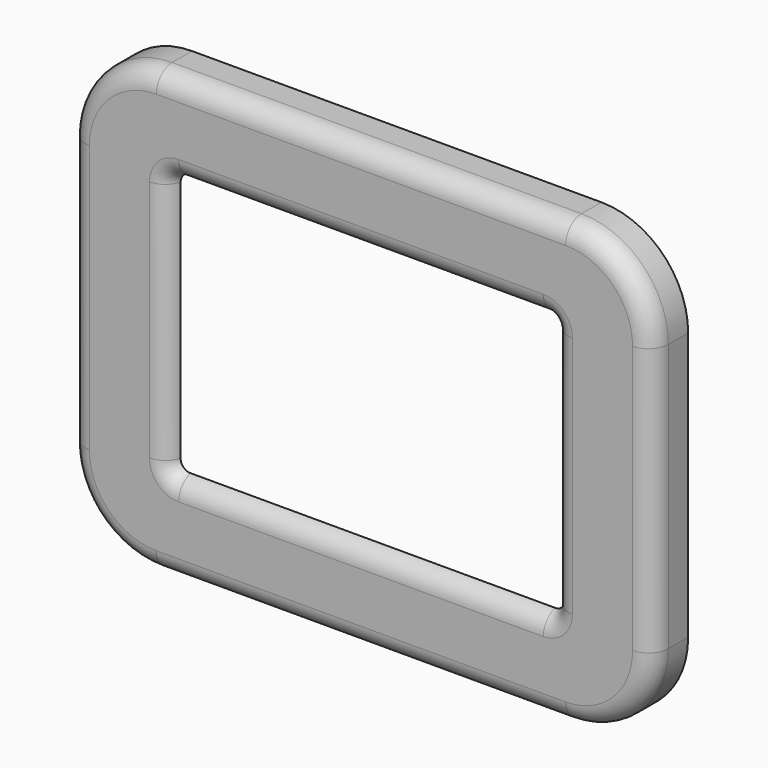
from build123d import *

# Parameters (mm, degrees)
F0_W         = 235
F0_H         = 178
F0_W_2       = 207
F0_H_2       = 156
F0_W_3       = 155
F0_H_3       = 106
F1_DEPTH     = 18
F2_DEPTH     = 12
F3_R         = 35
F4_R         = 4
F5_T1_DEPTH  = 98
F5_T3_DEPTH  = 147
F5_T5_DEPTH  = 165
F5_T7_DEPTH  = 108
F5_T10_ANGLE = 90
F5_T12_ANGLE = 90
F5_T14_ANGLE = 90
F5_T16_ANGLE = 90
F5_T18_ANGLE = 90
F5_T20_ANGLE = 90
F5_T22_ANGLE = 90
F5_T24_ANGLE = 90
F6_SIZE      = 3
F7_R         = 1.5
F8_DEPTH     = 16


# Not quite as in the source:
# - a fillet or chamfer that OpenCascade refuses, or shapes differently, is made with other operations: its cross-section is extruded or revolved along the edge and cut away or added


with BuildPart() as f1:
    # F0 (on Front) → F1 (new body)
    with BuildSketch(Plane.XZ):
        Rectangle(F0_W, F0_H)
        Rectangle(F0_W_2, F0_H_2, mode=Mode.SUBTRACT)
        Rectangle(F0_W_2, F0_H_2)
        Rectangle(F0_W_3, F0_H_3, mode=Mode.SUBTRACT)
    extrude(amount=F1_DEPTH)

    # F0 (on Front) → F2 (cut)
    with BuildSketch(Plane.XZ):
        Rectangle(F0_W_2, F0_H_2)
        Rectangle(F0_W_3, F0_H_3, mode=Mode.SUBTRACT)
    extrude(amount=F2_DEPTH, mode=Mode.SUBTRACT)

    # F3
    f3_edges = [f1.edges().sort_by_distance(p)[0] for p in [
        (117.5, -9, 89),
        (-117.5, -9, 89),
        (117.5, -9, -89),
        (-117.5, -9, -89),
    ]]
    fillet(f3_edges, radius=F3_R)

    # F4
    f4_edges = [f1.edges().sort_by_distance(p)[0] for p in [
        (-77.5, -15, 53),
        (77.5, -15, 53),
        (77.5, -15, -53),
        (-77.5, -15, -53),
    ]]
    fillet(f4_edges, radius=F4_R)

    # F5: fillet of radius 8 on 16 edges, made by hand

    # F5_s2 → F5_t1 (cut)
    with BuildSketch(Plane.XY.offset(-49)):
        with BuildLine():
            ThreePointArc((-85.2459666924, -18), (-80.3469872068, -16.3245553203), (-77.5, -12))
            Line((-77.5, -12), (-77.5, -18))
            Line((-77.5, -18), (-85.2459666924, -18))
        make_face()
        with BuildLine():
            ThreePointArc((85.2459666924, -18), (80.3469872068, -16.3245553203), (77.5, -12))
            Line((77.5, -12), (77.5, -18))
            Line((77.5, -18), (85.2459666924, -18))
        make_face()
    extrude(amount=F5_T1_DEPTH, mode=Mode.SUBTRACT)

    # F5_s4 → F5_t3 (cut)
    with BuildSketch(Plane.YZ.offset(-73.5)):
        with BuildLine():
            ThreePointArc((-18, -60.7459666924), (-16.3245553203, -55.8469872068), (-12, -53))
            Line((-12, -53), (-18, -53))
            Line((-18, -53), (-18, -60.7459666924))
        make_face()
        with BuildLine():
            ThreePointArc((-18, 60.7459666924), (-16.3245553203, 55.8469872068), (-12, 53))
            Line((-12, 53), (-18, 53))
            Line((-18, 53), (-18, 60.7459666924))
        make_face()
    extrude(amount=F5_T3_DEPTH, mode=Mode.SUBTRACT)

    # F5_s6 → F5_t5 (cut)
    with BuildSketch(Plane.YZ.offset(-82.5)):
        with BuildLine():
            ThreePointArc((-18, -81), (-15.6568542495, -86.6568542495), (-10, -89))
            Line((-10, -89), (-18, -89))
            Line((-18, -89), (-18, -81))
        make_face()
        with BuildLine():
            ThreePointArc((-18, 81), (-15.6568542495, 86.6568542495), (-10, 89))
            Line((-10, 89), (-18, 89))
            Line((-18, 89), (-18, 81))
        make_face()
    extrude(amount=F5_T5_DEPTH, mode=Mode.SUBTRACT)

    # F5_s8 → F5_t7 (cut)
    with BuildSketch(Plane.XY.offset(-54)):
        with BuildLine():
            ThreePointArc((-109.5, -18), (-115.1568542495, -15.6568542495), (-117.5, -10))
            Line((-117.5, -10), (-117.5, -18))
            Line((-117.5, -18), (-109.5, -18))
        make_face()
        with BuildLine():
            ThreePointArc((109.5, -18), (115.1568542495, -15.6568542495), (117.5, -10))
            Line((117.5, -10), (117.5, -18))
            Line((117.5, -18), (109.5, -18))
        make_face()
    extrude(amount=F5_T7_DEPTH, mode=Mode.SUBTRACT)

    # F5_s9 → F5_t10 (revolve, cut)
    with BuildSketch(Plane.XY.offset(-49)):
        with BuildLine():
            ThreePointArc((-85.2459666924, -18), (-80.3469872068, -16.3245553203), (-77.5, -12))
            Line((-77.5, -12), (-77.5, -18))
            Line((-77.5, -18), (-85.2459666924, -18))
        make_face()
    revolve(axis=Axis((-73.5, -18, -49), (0, -1, 0)), revolution_arc=F5_T10_ANGLE, mode=Mode.SUBTRACT)

    # F5_s11 → F5_t12 (revolve, cut)
    with BuildSketch(Plane.XY.offset(49)):
        with BuildLine():
            ThreePointArc((-85.2459666924, -18), (-80.3469872068, -16.3245553203), (-77.5, -12))
            Line((-77.5, -12), (-77.5, -18))
            Line((-77.5, -18), (-85.2459666924, -18))
        make_face()
    revolve(axis=Axis((-73.5, -18, 49), (0, 1, 0)), revolution_arc=F5_T12_ANGLE, mode=Mode.SUBTRACT)

    # F5_s13 → F5_t14 (revolve, cut)
    with BuildSketch(Plane.XY.offset(-49)):
        with BuildLine():
            ThreePointArc((85.2459666924, -18), (80.3469872068, -16.3245553203), (77.5, -12))
            Line((77.5, -12), (77.5, -18))
            Line((77.5, -18), (85.2459666924, -18))
        make_face()
    revolve(axis=Axis((73.5, -18, -49), (0, 1, 0)), revolution_arc=F5_T14_ANGLE, mode=Mode.SUBTRACT)

    # F5_s15 → F5_t16 (revolve, cut)
    with BuildSketch(Plane.YZ.offset(73.5)):
        with BuildLine():
            ThreePointArc((-18, 60.7459666924), (-16.3245553203, 55.8469872068), (-12, 53))
            Line((-12, 53), (-18, 53))
            Line((-18, 53), (-18, 60.7459666924))
        make_face()
    revolve(axis=Axis((73.5, -18, 49), (0, 1, 0)), revolution_arc=F5_T16_ANGLE, mode=Mode.SUBTRACT)

    # F5_s17 → F5_t18 (revolve, cut)
    with BuildSketch(Plane.YZ.offset(-82.5)):
        with BuildLine():
            ThreePointArc((-18, -81), (-15.6568542495, -86.6568542495), (-10, -89))
            Line((-10, -89), (-18, -89))
            Line((-18, -89), (-18, -81))
        make_face()
    revolve(axis=Axis((-82.5, -18, -54), (0, 1, 0)), revolution_arc=F5_T18_ANGLE, mode=Mode.SUBTRACT)

    # F5_s19 → F5_t20 (revolve, cut)
    with BuildSketch(Plane.YZ.offset(82.5)):
        with BuildLine():
            ThreePointArc((-18, -81), (-15.6568542495, -86.6568542495), (-10, -89))
            Line((-10, -89), (-18, -89))
            Line((-18, -89), (-18, -81))
        make_face()
    revolve(axis=Axis((82.5, -18, -54), (0, -1, 0)), revolution_arc=F5_T20_ANGLE, mode=Mode.SUBTRACT)

    # F5_s21 → F5_t22 (revolve, cut)
    with BuildSketch(Plane.XY.offset(54)):
        with BuildLine():
            ThreePointArc((-109.5, -18), (-115.1568542495, -15.6568542495), (-117.5, -10))
            Line((-117.5, -10), (-117.5, -18))
            Line((-117.5, -18), (-109.5, -18))
        make_face()
    revolve(axis=Axis((-82.5, -18, 54), (0, 1, 0)), revolution_arc=F5_T22_ANGLE, mode=Mode.SUBTRACT)

    # F5_s23 → F5_t24 (revolve, cut)
    with BuildSketch(Plane.XY.offset(54)):
        with BuildLine():
            ThreePointArc((109.5, -18), (115.1568542495, -15.6568542495), (117.5, -10))
            Line((117.5, -10), (117.5, -18))
            Line((117.5, -18), (109.5, -18))
        make_face()
    revolve(axis=Axis((82.5, -18, 54), (0, -1, 0)), revolution_arc=F5_T24_ANGLE, mode=Mode.SUBTRACT)

    # F6
    f6_edges = [f1.edges().sort_by_distance(p)[0] for p in [
        (-103.5, -6, -78),
        (103.5, -6, -78),
        (-103.5, -6, 78),
        (103.5, -6, 78),
    ]]
    chamfer(f6_edges, length=F6_SIZE)

    # F7 (on face) → F8 (join)
    with BuildSketch(Plane.XZ):
        with Locations((-103.5, -30)):
            Circle(F7_R)
        with Locations((-103.5, 30)):
            Circle(F7_R)
        with Locations((103.5, -30)):
            Circle(F7_R)
        with Locations((103.5, 30)):
            Circle(F7_R)
    extrude(amount=F8_DEPTH)


solid = f1.part
